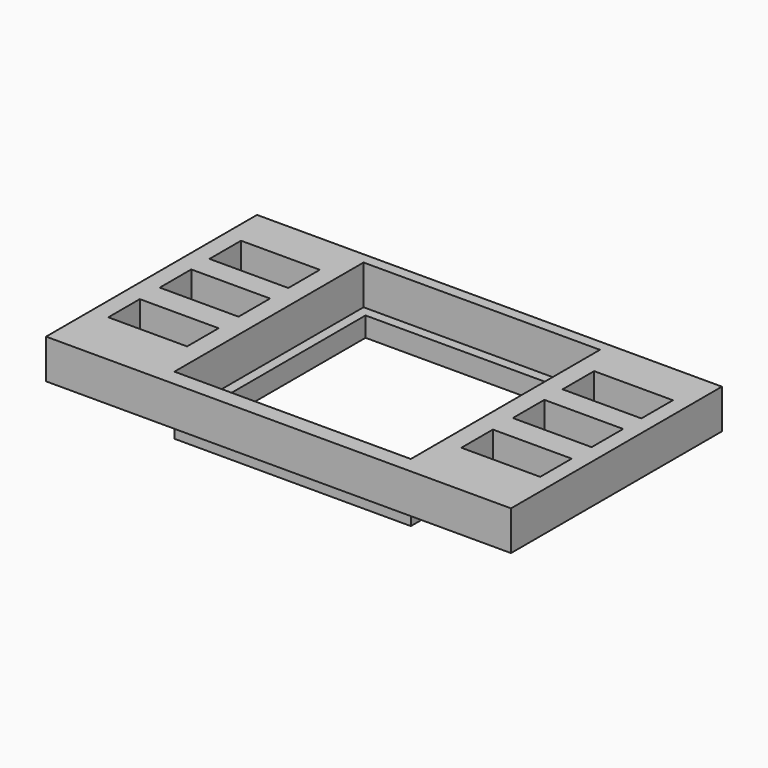
from build123d import *

# Parameters (mm, degrees)
F0_W     = 299.72
F0_H     = 169.9631744818
F3_DEPTH = 25.4
F1_W     = 50.8
F1_H     = 25.4
F4_DEPTH = 25.4
F2_W     = 152.4
F2_H     = 152.4
F2_W_2   = 139.7
F2_H_2   = 139.7
F5_DEPTH = 25.4
F6_DEPTH = 12.7


# Not quite as in the source:
# - a feature of the source that left no trace in its solid (it failed there, or was rolled back) is left out


with BuildPart() as f3:
    # F0 (on Top) → F3 (new body)
    with BuildSketch(Plane.XY):
        with Locations((-0.6489809602, -1.7615165561)):
            Rectangle(F0_W, F0_H)
    extrude(amount=F3_DEPTH)

    # F1 (on face) → F4 (cut)
    with BuildSketch(Plane.XY):
        with Locations((113.8091359086, 43.5188937416)):
            Rectangle(F1_W, F1_H)
        with Locations((113.8091359086, 3.428083711)):
            Rectangle(F1_W, F1_H)
        with Locations((113.8091359086, -38.0356973421)):
            Rectangle(F1_W, F1_H)
        with Locations((-113.8091359086, 43.5188937416)):
            Rectangle(F1_W, F1_H)
        with Locations((-113.8091359086, 3.428083711)):
            Rectangle(F1_W, F1_H)
        with Locations((-113.8091359086, -38.0356973421)):
            Rectangle(F1_W, F1_H)
    extrude(amount=F4_DEPTH, mode=Mode.SUBTRACT)

    # F2 (on Top) → F5 (cut)
    with BuildSketch(Plane.XY):
        Rectangle(F2_W, F2_H)
        Rectangle(F2_W_2, F2_H_2, mode=Mode.SUBTRACT)
        Rectangle(F2_W_2, F2_H_2)
    extrude(amount=F5_DEPTH, mode=Mode.SUBTRACT)


with BuildPart() as f6:
    # F2 (on Top) → F6 (new body)
    with BuildSketch(Plane.XY):
        Rectangle(F2_W, F2_H)
        Rectangle(F2_W_2, F2_H_2, mode=Mode.SUBTRACT)
    extrude(amount=-F6_DEPTH)


solid = Compound([f3.part, f6.part])
